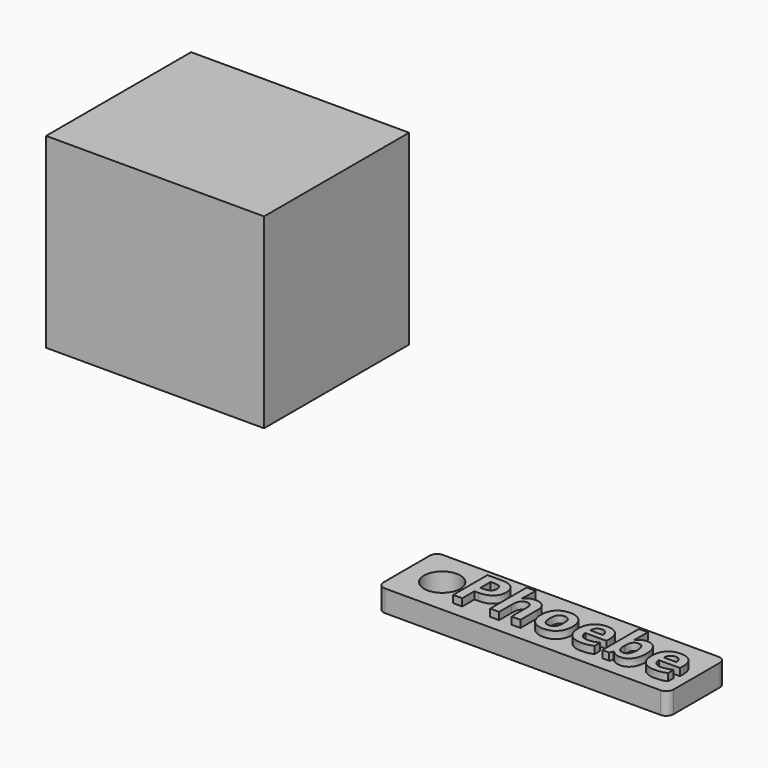
from build123d import *

# Parameters (mm, degrees)
F0_W         = 40
F0_H         = 10
F0_R         = 2.5
F1_DEPTH     = 3
F2_TEXT_SIZE = 8.2873851295
F3_DEPTH     = 1
F4_R         = 1
F5_W         = 30.0630871207
F5_H         = 25.7270652801
F6_DEPTH     = 25


# Not quite as in the source:
# - Text() gives the source's letters only with a copy of the font that has no kerning and outlines rounded to 1/6400 em; it was checked with that copy


with BuildPart() as f1:
    # F0 (on Top) → F1 (new body)
    with BuildSketch(Plane.XY):
        Rectangle(F0_W, F0_H)
        with Locations((-15.0961216106, 0)):
            Circle(F0_R, mode=Mode.SUBTRACT)
    extrude(amount=F1_DEPTH)

    # F2 (on face) → F3 (join)
    with BuildSketch(Plane.XY.offset(3)):
        with Locations((-11.8574339504, -3.0901126025)):
            Text('Phoebe', F2_TEXT_SIZE, font='Open Sans', font_style=FontStyle.BOLD, text_align=(TextAlign.LEFT, TextAlign.BOTTOM))
    extrude(amount=F3_DEPTH)

    # F4
    f4_edges = [f1.edges().sort_by_distance(p)[0] for p in [
        (-20, -5, 1.5),
        (-20, 5, 1.5),
        (20, -5, 1.5),
        (20, 5, 1.5),
    ]]
    fillet(f4_edges, radius=F4_R)


with BuildPart() as f6:
    # F5 (on Front) → F6 (new body)
    with BuildSketch(Plane.XZ):
        with Locations((-34.6881812438, 43.2156873867)):
            Rectangle(F5_W, F5_H)
    extrude(amount=F6_DEPTH)


solid = Compound([f1.part, f6.part])
